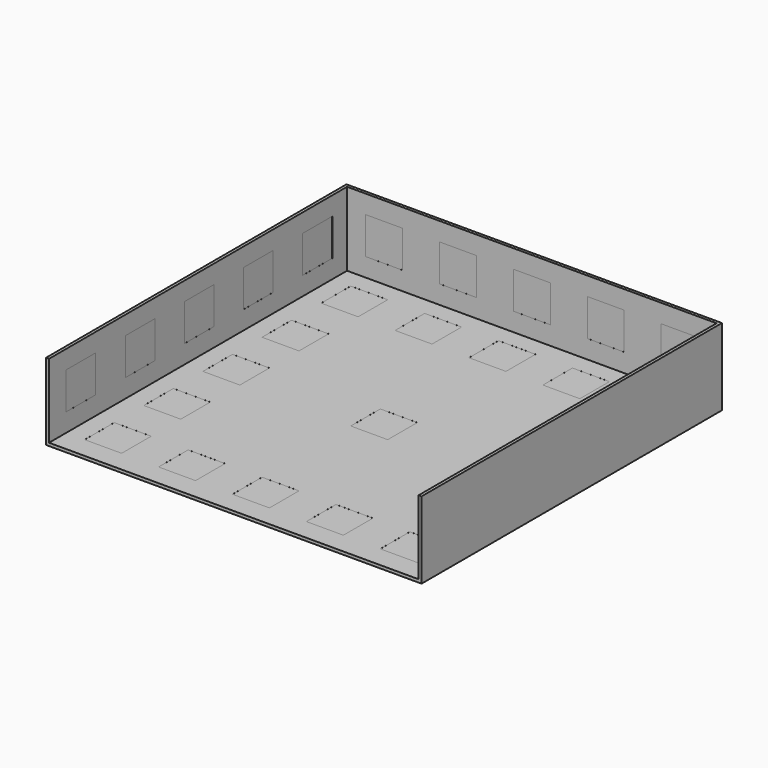
from build123d import *

# Parameters (mm, degrees)
F1_W            = 1250
F1_H            = 1250
F2_DEPTH        = 10
F0_W            = 125
F0_H            = 125
F3_DEPTH        = 0.1
F4_W            = 1270
F4_H            = 1270
F4_W_2          = 1250
F4_H_2          = 1250
F5_DEPTH        = 260
F6_W            = 125
F6_H            = 125
F7_DEPTH        = 0.1
F7_COPIES_COUNT = 3
F7_COPIES_ANGLE = 180
F9_W            = 1250
F9_H            = 10
F10_DEPTH       = 250


# Not quite as in the source:
# - a pattern or mirror of a feature is missing from the dataset's text; its kind, count and spacing are read off the source's solid


with BuildPart() as f2:
    # F1 (on Top) → F2 (new body)
    with BuildSketch(Plane.XY):
        Rectangle(F1_W, F1_H)
    extrude(amount=-F2_DEPTH)

    # F0 (on Top) → F3 (cut)
    with BuildSketch(Plane.XY):
        with Locations((-500, 500)):
            Rectangle(F0_W, F0_H)
        with Locations((-250, 500)):
            Rectangle(F0_W, F0_H)
        with Locations((0, 500)):
            Rectangle(F0_W, F0_H)
        with Locations((250, 500)):
            Rectangle(F0_W, F0_H)
        with Locations((500, 500)):
            Rectangle(F0_W, F0_H)
        with Locations((-500, 250)):
            Rectangle(F0_W, F0_H)
        with Locations((-500, 0)):
            Rectangle(F0_W, F0_H)
        with Locations((-500, -250)):
            Rectangle(F0_W, F0_H)
        with Locations((-500, -500)):
            Rectangle(F0_W, F0_H)
        with Locations((250, -500)):
            Rectangle(F0_W, F0_H)
        with Locations((500, -500)):
            Rectangle(F0_W, F0_H)
        with Locations((500, 250)):
            Rectangle(F0_W, F0_H)
        with Locations((-250, -500)):
            Rectangle(F0_W, F0_H)
        with Locations((500, 0)):
            Rectangle(F0_W, F0_H)
        with Locations((0, -500)):
            Rectangle(F0_W, F0_H)
        with Locations((500, -250)):
            Rectangle(F0_W, F0_H)
        Rectangle(F0_W, F0_H)
    extrude(amount=-F3_DEPTH, mode=Mode.SUBTRACT)

    # F4 (on face) → F5 (join)
    with BuildSketch(Plane(origin=(0, 0, -10), x_dir=(1, 0, 0), z_dir=(0, 0, -1))):
        Rectangle(F4_W, F4_H)
        Rectangle(F4_W_2, F4_H_2, mode=Mode.SUBTRACT)
    extrude(amount=-F5_DEPTH)

    # F6 (on face) → F7 (cut)
    with BuildSketch(Plane.YZ.offset(-625)):
        with Locations((-499.9999926, 125.0000074)):
            Rectangle(F6_W, F6_H)
        with Locations((-249.9999926, 125.0000074)):
            Rectangle(F6_W, F6_H)
        with Locations((7.4e-06, 125.0000074)):
            Rectangle(F6_W, F6_H)
        with Locations((250.0000074, 125.0000074)):
            Rectangle(F6_W, F6_H)
        with Locations((500.0000074, 125.0000074)):
            Rectangle(F6_W, F6_H)
    f7 = extrude(amount=-F7_DEPTH, mode=Mode.SUBTRACT)

    # F7_copies: F7 ×3 about axis
    f7_copies_axis = Axis((0, 0, 0), (0, 0, -1))
    for i in range(1, F7_COPIES_COUNT):
        add(f7.rotate(f7_copies_axis, i * F7_COPIES_ANGLE / (F7_COPIES_COUNT - 1)), mode=Mode.SUBTRACT)

    # F9 (on face) → F10 (cut, through all)
    with BuildSketch(Plane.XY.offset(250)):
        with Locations((0, -630)):
            Rectangle(F9_W, F9_H)
    extrude(amount=-F10_DEPTH, mode=Mode.SUBTRACT)


solid = f2.part
